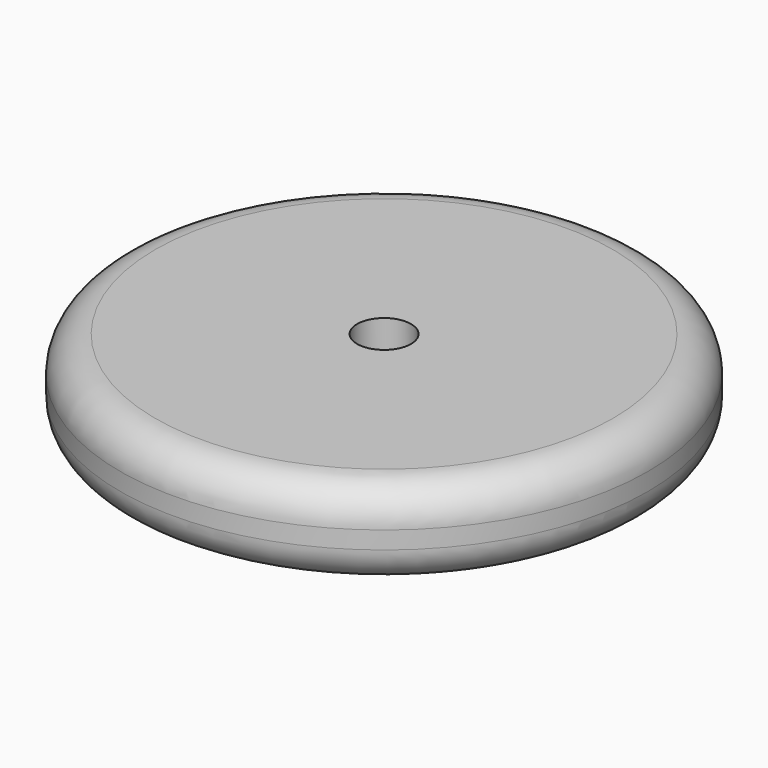
from build123d import *

# Parameters (mm, degrees)
F0_R     = 11.43
F1_DEPTH = 1.905
F2_R     = 1.1684
F3_DEPTH = 25.4
F4_R     = 1.524


with BuildPart() as f1:
    # F0 (on Top) → F1 (new body, symmetric)
    with BuildSketch(Plane.XY):
        Circle(F0_R)
    extrude(amount=F1_DEPTH, both=True)

    # F2 (on face) → F3 (cut)
    with BuildSketch(Plane(origin=(0, 0, -1.905), x_dir=(1, 0, 0), z_dir=(0, 0, -1))):
        Circle(F2_R)
    extrude(amount=-F3_DEPTH, mode=Mode.SUBTRACT)

    # F4
    f4_edges = [f1.edges().sort_by_distance(p)[0] for p in [
        (-11.43, 0, 1.905),
        (-11.43, 0, -1.905),
    ]]
    fillet(f4_edges, radius=F4_R)


solid = f1.part
